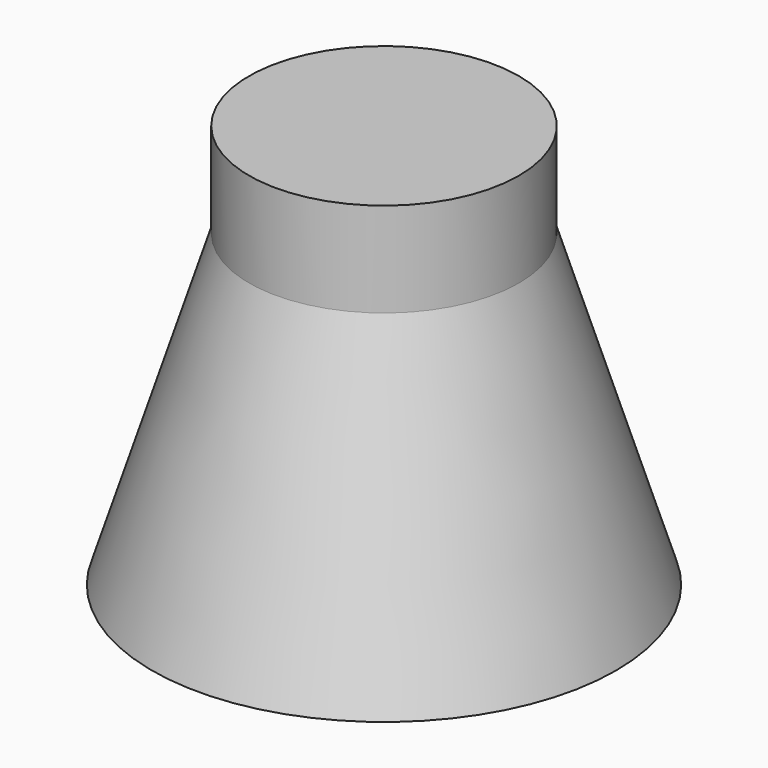
from build123d import *

# Parameters (mm, degrees)
F2_TEXT_SIZE = 7.1819108497
F3_DEPTH     = 1.00000054


# Not quite as in the source:
# - Text() gives the source's letters only with a copy of the font that has no kerning and outlines rounded to 1/6400 em; it was checked with that copy


with BuildPart() as f1:
    # F0 (on Front) → F1 (revolve)
    with BuildSketch(Plane.XZ):
        Polygon((0, 1.49999954), (0, 0), (6.35, 0), (6.35, -3.999992), (7.85, -3.999992), (7.85, 1.49999954), align=None)
        Polygon((7.85, -3.999992), (6.35, -3.999992), (12, -22.0000068), (13.5, -22.0000068), align=None)
    revolve(axis=Axis((0, 0, -11.0000034), (0, 0, -1)))

    # F2 (on face) → F3 (join)
    with BuildSketch(Plane(origin=(0, 0, 0), x_dir=(1, 0, 0), z_dir=(0, 0, -1))):
        with Locations((-4.8863461707, -2.4018250406)):
            Text('CN', F2_TEXT_SIZE, font='Open Sans', text_align=(TextAlign.LEFT, TextAlign.BOTTOM))
    extrude(amount=F3_DEPTH)


solid = f1.part
